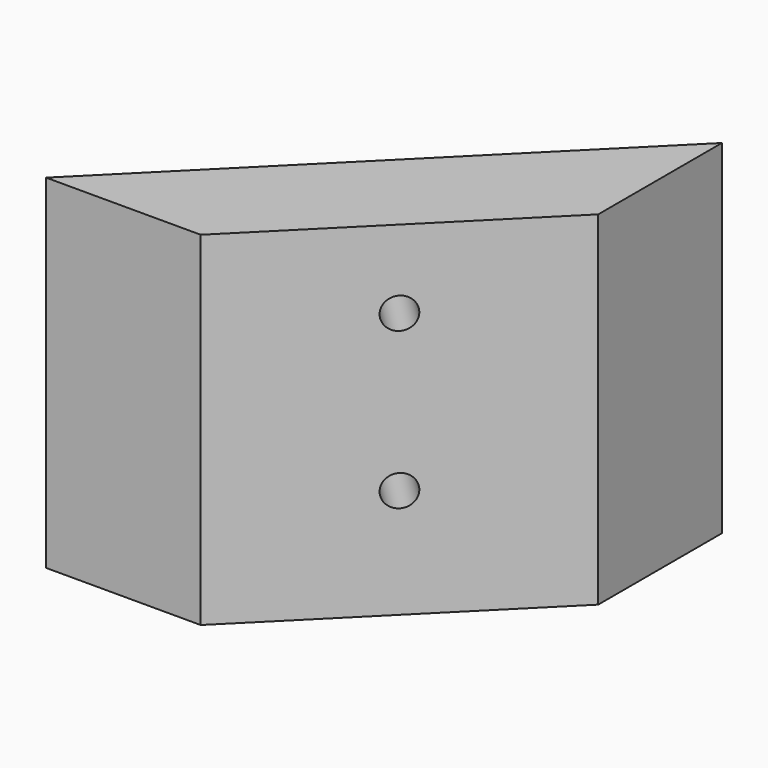
from build123d import *

# Parameters (mm, degrees)
F1_DEPTH = 34.925
F2_SIZE  = 22.22499
F3_SIZE  = 22.22499
F5_D     = 6.35
F6_D     = 6.35


# Not quite as in the source:
# - a fillet or chamfer is up to 0.001 mm smaller than in the source, because OpenCascade refuses the exact size


with BuildPart() as f1:
    # F0 (on Top) → F1 (new body, symmetric)
    with BuildSketch(Plane.XY):
        Polygon((-46.0238126205, -30.3083644086), (-30.3083644086, -46.0238126205), (46.0238126205, 30.3083644086), (30.3083644086, 46.0238126205), align=None)
    extrude(amount=F1_DEPTH, both=True)

    # F2 (size 22.225 in the source; OpenCascade refuses exactly that, so slightly less here)
    f2_edges = [f1.edges().sort_by_distance(p)[0] for p in [
        (46.023813, 30.308364, 0),
    ]]
    chamfer(f2_edges, length=F2_SIZE)

    # F3 (size 22.225 in the source; OpenCascade refuses exactly that, so slightly less here)
    f3_edges = [f1.edges().sort_by_distance(p)[0] for p in [
        (-30.308364, -46.023813, 0),
    ]]
    chamfer(f3_edges, length=F3_SIZE)

    # F5 (through all)
    with Locations(Plane(origin=(7.8577241059, -7.8577241059, 0), x_dir=(0.7071067812, 0.7071067812, 0), z_dir=(0.7071067812, -0.7071067812, 0))):
        with Locations((0, 19.05)):
            Hole(F5_D / 2)

    # F6 (through all)
    with Locations(Plane(origin=(7.8577241059, -7.8577241059, 0), x_dir=(0.7071067812, 0.7071067812, 0), z_dir=(0.7071067812, -0.7071067812, 0))):
        with Locations((0, -12.7)):
            Hole(F6_D / 2)


solid = f1.part
